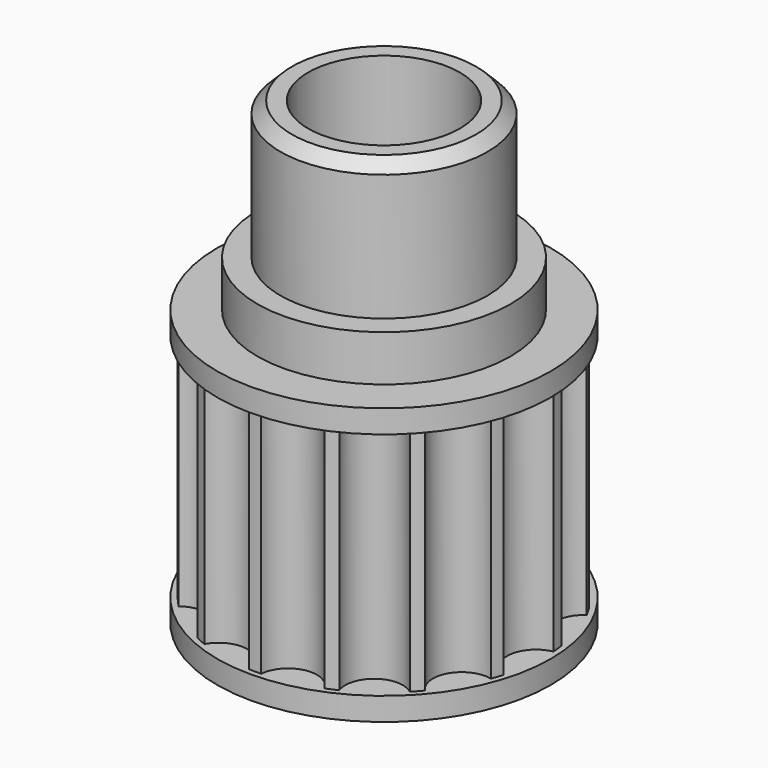
from build123d import *

# Parameters (mm, degrees)
F0_R            = 7.25
F1_DEPTH        = 1
F2_R            = 7.25
F3_DEPTH        = 11
F4_R            = 1.25
F5_DEPTH        = 10
F5_COPIES_COUNT = 15
F6_R            = 7.25
F6_R_2          = 7
F7_DEPTH        = 10
F8_R            = 5.5
F9_DEPTH        = 2
F10_R           = 4.5
F11_DEPTH       = 6
F12_R           = 3.3
F13_DEPTH       = 25
F14_SIZE        = 0.5


# Not quite as in the source:
# - a pattern or mirror of a feature is missing from the dataset's text; its kind, count and spacing are read off the source's solid


with BuildPart() as f1:
    # F0 (on Top) → F1 (new body)
    with BuildSketch(Plane.XY):
        Circle(F0_R)
    extrude(amount=F1_DEPTH)


with BuildPart() as f3:
    # F2 (on face) → F3 (new body)
    with BuildSketch(Plane.XY.offset(1)):
        Circle(F2_R)
    extrude(amount=F3_DEPTH)

    # F4 (on face) → F5 (cut)
    with BuildSketch(Plane(origin=(0, 0, 1), x_dir=(1, 0, 0), z_dir=(0, 0, -1))):
        with Locations((0, -7.25)):
            Circle(F4_R)
    f5 = extrude(amount=-F5_DEPTH, mode=Mode.SUBTRACT)

    # F5_copies: F5 ×15 about axis
    f5_copies_axis = Axis((0, 0, 0), (0, 0, 1))
    for i in range(1, F5_COPIES_COUNT):
        add(f5.rotate(f5_copies_axis, i * 360 / F5_COPIES_COUNT), mode=Mode.SUBTRACT)

    # F6 (on face) → F7 (cut)
    with BuildSketch(Plane(origin=(0, 0, 1), x_dir=(1, 0, 0), z_dir=(0, 0, -1))):
        Circle(F6_R)
        Circle(F6_R_2, mode=Mode.SUBTRACT)
    extrude(amount=-F7_DEPTH, mode=Mode.SUBTRACT)

    # F8 (on face) → F9 (join)
    with BuildSketch(Plane.XY.offset(12)):
        Circle(F8_R)
    extrude(amount=F9_DEPTH)

    # F10 (on face) → F11 (join)
    with BuildSketch(Plane.XY.offset(14)):
        Circle(F10_R)
    extrude(amount=F11_DEPTH)


with BuildPart() as f13_tool:
    # F12 (on face) → F13 (new body)
    with BuildSketch(Plane.XY.offset(20)):
        Circle(F12_R)
    extrude(amount=-F13_DEPTH)


with BuildPart() as f1_1:
    add(f1.part)

    # F13: cut by f13_tool
    add(f13_tool.part, mode=Mode.SUBTRACT)


with BuildPart() as f3_1:
    add(f3.part)

    # F13: cut by f13_tool
    add(f13_tool.part, mode=Mode.SUBTRACT)

    # F14
    f14_edges = [f3_1.edges().sort_by_distance(p)[0] for p in [
        (-4.5, 0, 20),
    ]]
    chamfer(f14_edges, length=F14_SIZE)


solid = Compound([f1_1.part, f3_1.part])
